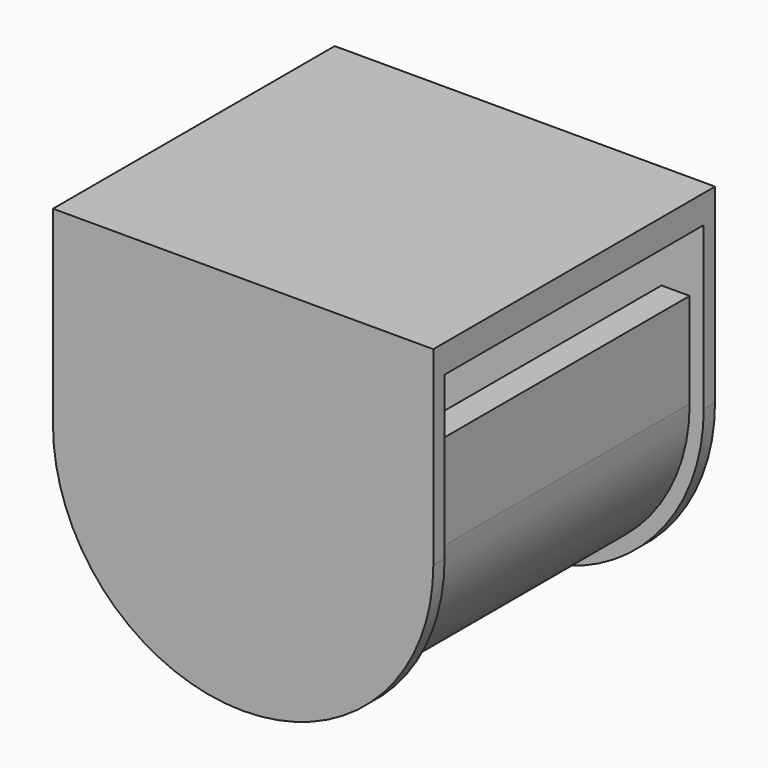
from build123d import *

# Parameters (mm, degrees)
F0_W     = 2
F0_H     = 2
F0_W_2   = 1
F0_W_3   = 21
F1_DEPTH = 25
F2_DEPTH = 1
F3_START = 24
F3_DEPTH = 1
F4_W     = 23
F4_H     = 4.75
F5_DEPTH = 25


with BuildPart() as f1:
    # F0 (on Front) → F1 (new body)
    with BuildSketch(Plane.XZ):
        with BuildLine():
            Line((-12.4285714286, 13.5171716937), (-14.4285714286, 13.5171716937))
            Line((-14.4285714286, 13.5171716937), (-14.4285714286, 2.0171716937))
            ThreePointArc((-14.4285714286, 2.0171716937), (-1.9285714286, -10.4828283063), (10.5714285714, 2.0171716937))
            Line((10.5714285714, 2.0171716937), (10.5714285714, 13.5171716937))
            Line((10.5714285714, 13.5171716937), (8.5714285714, 13.5171716937))
            Line((8.5714285714, 13.5171716937), (8.5714285714, 2.0171716937))
            ThreePointArc((8.5714285714, 2.0171716937), (-1.9285714286, -8.4828283063), (-12.4285714286, 2.0171716937))
            Line((-12.4285714286, 2.0171716937), (-12.4285714286, 13.5171716937))
        make_face()
        with Locations((9.5714285714, 14.5171716937)):
            Rectangle(F0_W, F0_H)
        with Locations((-13.4285714286, 14.5171716937)):
            Rectangle(F0_W, F0_H)
        with Locations((-14.9285714286, 14.5171716937)):
            Rectangle(F0_W_2, F0_H)
        with Locations((-1.9285714286, 14.5171716937)):
            Rectangle(F0_W_3, F0_H)
        with Locations((11.0714285714, 14.5171716937)):
            Rectangle(F0_W_2, F0_H)
    extrude(amount=F1_DEPTH)

    # F0 (on Front) → F2 (join)
    with BuildSketch(Plane.XZ):
        with BuildLine():
            Line((-14.4285714286, 13.5171716937), (-15.4285714286, 13.5171716937))
            Line((-15.4285714286, 13.5171716937), (-15.4285714286, 2.0171716937))
            ThreePointArc((-15.4285714286, 2.0171716937), (-11.4745129746, -7.5287698523), (-1.9285714286, -11.4828283063))
            ThreePointArc((-1.9285714286, -11.4828283063), (7.6173701174, -7.5287698523), (11.5714285714, 2.0171716937))
            Line((11.5714285714, 2.0171716937), (11.5714285714, 13.5171716937))
            Line((11.5714285714, 13.5171716937), (10.5714285714, 13.5171716937))
            Line((10.5714285714, 13.5171716937), (10.5714285714, 2.0171716937))
            ThreePointArc((10.5714285714, 2.0171716937), (-1.9285714286, -10.4828283063), (-14.4285714286, 2.0171716937))
            Line((-14.4285714286, 2.0171716937), (-14.4285714286, 13.5171716937))
        make_face()
        with BuildLine():
            Line((-12.4285714286, 13.5171716937), (-14.4285714286, 13.5171716937))
            Line((-14.4285714286, 13.5171716937), (-14.4285714286, 2.0171716937))
            ThreePointArc((-14.4285714286, 2.0171716937), (-1.9285714286, -10.4828283063), (10.5714285714, 2.0171716937))
            Line((10.5714285714, 2.0171716937), (10.5714285714, 13.5171716937))
            Line((10.5714285714, 13.5171716937), (8.5714285714, 13.5171716937))
            Line((8.5714285714, 13.5171716937), (8.5714285714, 2.0171716937))
            ThreePointArc((8.5714285714, 2.0171716937), (-1.9285714286, -8.4828283063), (-12.4285714286, 2.0171716937))
            Line((-12.4285714286, 2.0171716937), (-12.4285714286, 13.5171716937))
        make_face()
        with BuildLine():
            Line((8.5714285714, 13.5171716937), (-12.4285714286, 13.5171716937))
            Line((-12.4285714286, 13.5171716937), (-12.4285714286, 2.0171716937))
            ThreePointArc((-12.4285714286, 2.0171716937), (-1.9285714286, -8.4828283063), (8.5714285714, 2.0171716937))
            Line((8.5714285714, 2.0171716937), (8.5714285714, 13.5171716937))
        make_face()
    extrude(amount=F2_DEPTH)

    # F0 (on Front) → F3 (join)
    with BuildSketch(Plane.XZ.offset(F3_START)):
        with BuildLine():
            Line((-14.4285714286, 13.5171716937), (-15.4285714286, 13.5171716937))
            Line((-15.4285714286, 13.5171716937), (-15.4285714286, 2.0171716937))
            ThreePointArc((-15.4285714286, 2.0171716937), (-11.4745129746, -7.5287698523), (-1.9285714286, -11.4828283063))
            ThreePointArc((-1.9285714286, -11.4828283063), (7.6173701174, -7.5287698523), (11.5714285714, 2.0171716937))
            Line((11.5714285714, 2.0171716937), (11.5714285714, 13.5171716937))
            Line((11.5714285714, 13.5171716937), (10.5714285714, 13.5171716937))
            Line((10.5714285714, 13.5171716937), (10.5714285714, 2.0171716937))
            ThreePointArc((10.5714285714, 2.0171716937), (-1.9285714286, -10.4828283063), (-14.4285714286, 2.0171716937))
            Line((-14.4285714286, 2.0171716937), (-14.4285714286, 13.5171716937))
        make_face()
        with BuildLine():
            Line((-12.4285714286, 13.5171716937), (-14.4285714286, 13.5171716937))
            Line((-14.4285714286, 13.5171716937), (-14.4285714286, 2.0171716937))
            ThreePointArc((-14.4285714286, 2.0171716937), (-1.9285714286, -10.4828283063), (10.5714285714, 2.0171716937))
            Line((10.5714285714, 2.0171716937), (10.5714285714, 13.5171716937))
            Line((10.5714285714, 13.5171716937), (8.5714285714, 13.5171716937))
            Line((8.5714285714, 13.5171716937), (8.5714285714, 2.0171716937))
            ThreePointArc((8.5714285714, 2.0171716937), (-1.9285714286, -8.4828283063), (-12.4285714286, 2.0171716937))
            Line((-12.4285714286, 2.0171716937), (-12.4285714286, 13.5171716937))
        make_face()
        with BuildLine():
            Line((8.5714285714, 13.5171716937), (-12.4285714286, 13.5171716937))
            Line((-12.4285714286, 13.5171716937), (-12.4285714286, 2.0171716937))
            ThreePointArc((-12.4285714286, 2.0171716937), (-1.9285714286, -8.4828283063), (8.5714285714, 2.0171716937))
            Line((8.5714285714, 2.0171716937), (8.5714285714, 13.5171716937))
        make_face()
    extrude(amount=F3_DEPTH)

    # F4 (on face) → F5 (cut, through all)
    with BuildSketch(Plane(origin=(-14.4285714286, 0, 0), x_dir=(0, -1, 0), z_dir=(-1, 0, 0))):
        with Locations((12.5, 11.1421716937)):
            Rectangle(F4_W, F4_H)
    extrude(amount=-F5_DEPTH, mode=Mode.SUBTRACT)


solid = f1.part
